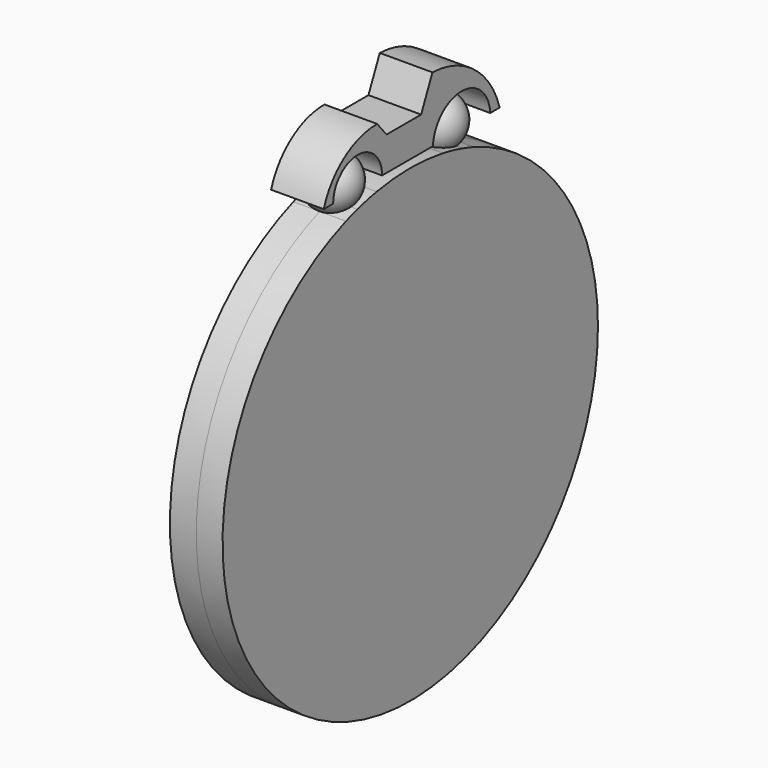
from build123d import *

# Parameters (mm, degrees)
F2_DEPTH      = 10
F2_DEPTH_BACK = 10
F3_DEPTH      = 10
F3_DEPTH_BACK = 10


with BuildPart() as f1:
    # F0 (on Right) → F1 (revolve)
    with BuildSketch(Plane.YZ):
        with BuildLine():
            Line((-38.7784093618, 0), (-28.7784093618, 0))
            ThreePointArc((-28.7784093618, 0), (-38.7784093618, 10), (-48.7784093618, 0))
            Line((-48.7784093618, 0), (-38.7784093618, 0))
        make_face()
    revolve(axis=Axis((0, -14.0198855661, 0), (0, 1, 0)))


with BuildPart() as f1b:
    # F0 (on Right) → F1, piece 2 (revolve)
    with BuildSketch(Plane.YZ):
        with BuildLine():
            ThreePointArc((20.7386382297, 0), (10.7386382297, 10), (0.7386382297, 0))
            Line((0.7386382297, 0), (10.7386382297, 0))
            Line((10.7386382297, 0), (20.7386382297, 0))
        make_face()
    revolve(axis=Axis((0, -14.0198855661, 0), (0, 1, 0)))


with BuildPart() as f2:
    # F0 (on Right) → F2 (new body, two sides)
    with BuildSketch(Plane.YZ) as f2_sk:
        with BuildLine():
            ThreePointArc((-50.4119358957, 0), (-38.8033691557, 11.6107195707), (-27.1948024158, 0))
            Line((-27.1948024158, 0), (-3.0528949055, 0))
            ThreePointArc((-3.0528949055, 0), (10.5545190422, 12.8352438109), (24.16193299, 0))
            Line((24.16193299, 0), (28.6363661289, 0))
            ThreePointArc((28.6363661289, 0), (16.6846966655, 17.5450922675), (-3.2812512945, 24.7585233301))
            Line((-3.2812512945, 24.7585233301), (-8.6505692452, 12.8267044201))
            Line((-8.6505692452, 12.8267044201), (-25.0568185002, 12.8267044201))
            Line((-25.0568185002, 12.8267044201), (-29.5312516391, 18.1960240006))
            ThreePointArc((-29.5312516391, 18.1960240006), (-45.1714995095, 13.2263526785), (-54.8863634467, 0))
            Line((-54.8863634467, 0), (-50.4119358957, 0))
        make_face()
    extrude(amount=F2_DEPTH)
    extrude(f2_sk.sketch, amount=-F2_DEPTH_BACK)


with BuildPart() as f3:
    # F0 (on Right) → F3 (new body, two sides)
    with BuildSketch(Plane.YZ) as f3_sk:
        with BuildLine():
            ThreePointArc((1.7100001057, -4.2992666382), (-14.0433656752, -2.9374034586), (-29.7894036735, -4.3815267585))
            ThreePointArc((-29.7894036735, -4.3815267585), (-36.1603319482, -9.6512004775), (-44.3209305081, -8.3234884119))
            ThreePointArc((-44.3209305081, -8.3234884119), (-64.9028354001, -165.0400861413), (75.2925169547, -92.0402916829))
            ThreePointArc((75.2925169547, -92.0402916829), (59.1058533817, -40.8293679595), (16.426865836, -8.2246013094))
            ThreePointArc((16.426865836, -8.2246013094), (8.1614985989, -9.662212548), (1.7100001057, -4.2992666382))
        make_face()
        with BuildLine():
            ThreePointArc((-44.3209305081, -8.3234884119), (-36.1603319482, -9.6512004775), (-29.7894036735, -4.3815267585))
            ThreePointArc((-29.7894036735, -4.3815267585), (-34.3927217868, -5.3468190964), (-38.9386899769, -6.5536745824))
            ThreePointArc((-38.9386899769, -6.5536745824), (-41.6438808141, -7.3957910072), (-44.3209305081, -8.3234884119))
        make_face()
        with BuildLine():
            ThreePointArc((11.1030079424, -6.4909653738), (6.4361818801, -5.2679250151), (1.7100001057, -4.2992666382))
            ThreePointArc((1.7100001057, -4.2992666382), (8.1614985989, -9.662212548), (16.426865836, -8.2246013094))
            ThreePointArc((16.426865836, -8.2246013094), (13.7785574006, -7.315955836), (11.1030079424, -6.4909653738))
        make_face()
    extrude(amount=F3_DEPTH)
    extrude(f3_sk.sketch, amount=-F3_DEPTH_BACK)


solid = Compound([f1.part, f1b.part, f2.part, f3.part])
